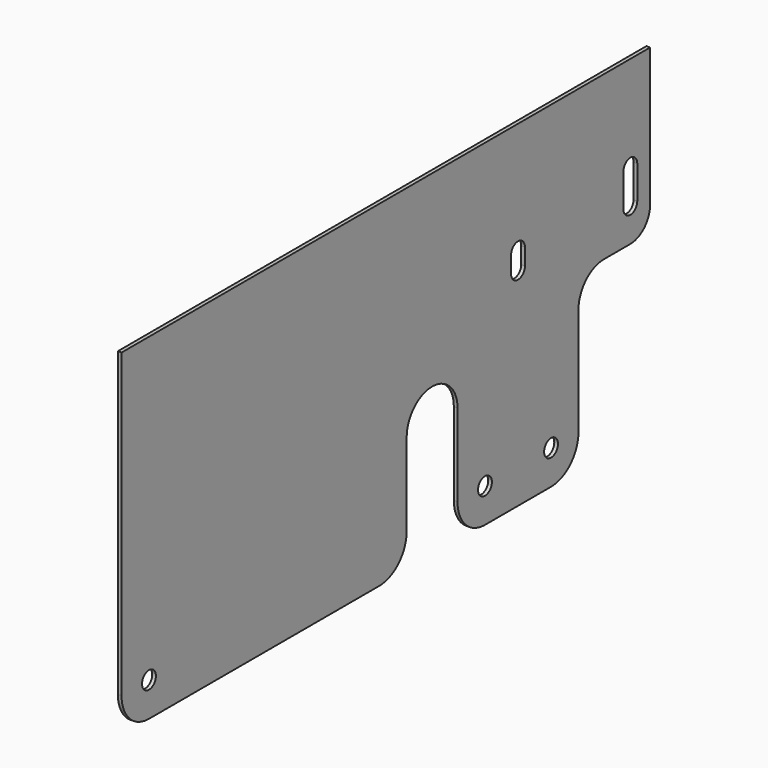
from build123d import *

# Parameters (mm, degrees)
F0_R     = 10.5
F1_DEPTH = 4.5


# Not quite as in the source:
# - a feature names something its author has since deleted; it is built from what else it names


with BuildPart() as f1:
    # F0 (on Right) → F1 (new body)
    with BuildSketch(Plane.YZ):
        with BuildLine():
            Line((-800, -79.2), (-800, -246.5))
            Line((-800, -246.5), (-800, -445))
            ThreePointArc((-800, -445), (-787.8449314192, -474.3449314192), (-758.5, -486.5))
            Line((-758.5, -486.5), (-410, -486.5))
            ThreePointArc((-410, -486.5), (-380.6550685808, -474.3449314192), (-368.5, -445))
            Line((-368.5, -445), (-368.5, -345))
            ThreePointArc((-368.5, -345), (-330, -306.5), (-291.5, -345))
            Line((-291.5, -345), (-291.5, -445))
            ThreePointArc((-291.5, -445), (-279.3449314192, -474.3449314192), (-250, -486.5))
            Line((-250, -486.5), (-150, -486.5))
            ThreePointArc((-150, -486.5), (-120.6550685808, -474.3449314192), (-108.5, -445))
            Line((-108.5, -445), (-108.5, -315))
            ThreePointArc((-108.5, -315), (-97.2236110757, -287.7763889243), (-70, -276.5))
            Line((-70, -276.5), (-30, -276.5))
            ThreePointArc((-30, -276.5), (-8.7867965644, -267.7132034356), (0, -246.5))
            Line((0, -246.5), (0, -79.2))
            Line((0, -79.2), (-800, -79.2))
        make_face()
        with Locations((-758.5, -445)):
            Circle(F0_R, mode=Mode.SUBTRACT)
        with Locations((-250, -445)):
            Circle(F0_R, mode=Mode.SUBTRACT)
        with Locations((-150, -445)):
            Circle(F0_R, mode=Mode.SUBTRACT)
        with BuildLine():
            ThreePointArc((-210.5, -215), (-200, -204.5), (-189.5, -215))
            Line((-189.5, -215), (-189.5, -235))
            ThreePointArc((-189.5, -235), (-200, -245.5), (-210.5, -235))
            Line((-210.5, -235), (-210.5, -215))
        make_face(mode=Mode.SUBTRACT)
        with BuildLine():
            ThreePointArc((-40.5, -195), (-30, -184.5), (-19.5, -195))
            Line((-19.5, -195), (-19.5, -235))
            ThreePointArc((-19.5, -235), (-30, -245.5), (-40.5, -235))
            Line((-40.5, -235), (-40.5, -195))
        make_face(mode=Mode.SUBTRACT)
    extrude(amount=F1_DEPTH)


solid = f1.part
